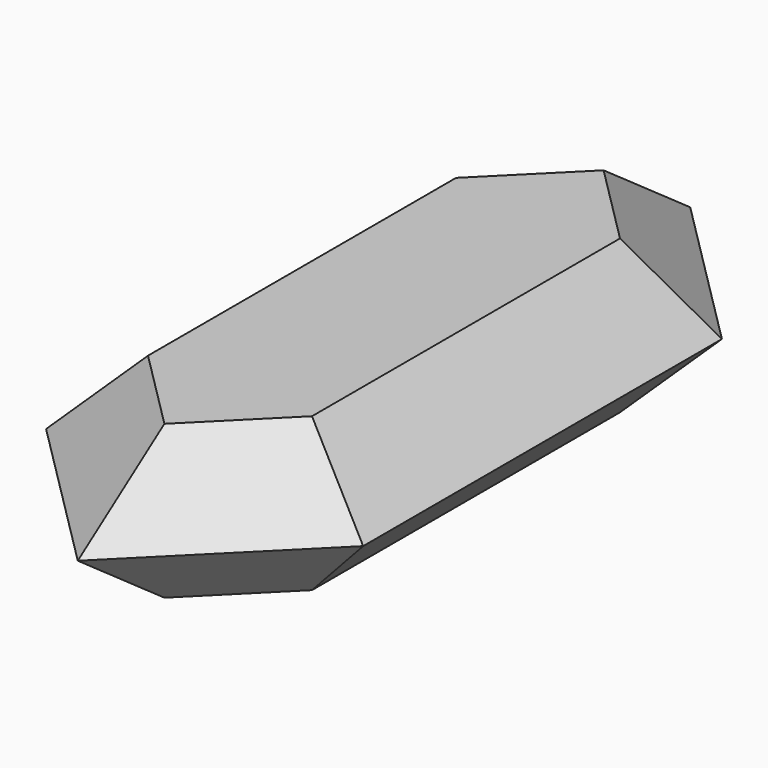
from build123d import *

# Parameters (mm, degrees)
F1_DEPTH = 6
F2_SIZE  = 2.99999


# Not quite as in the source:
# - a fillet or chamfer is up to 0.001 mm smaller than in the source, because OpenCascade refuses the exact size


with BuildPart() as f1:
    # F0 (on Top) → F1 (new body)
    with BuildSketch(Plane.XY):
        Polygon((-6.2132034356, 8.7867965644), (-6.2132034356, 0), (-6.2132034356, -8.7867965644), (0, -15), (6.2132034356, -8.7867965644), (6.2132034356, 0), (6.2132034356, 8.7867965644), (0, 15), align=None)
    extrude(amount=F1_DEPTH)

    # F2 (size 3 in the source; OpenCascade refuses exactly that, so slightly less here)
    f2_edges = [f1.edges().sort_by_distance(p)[0] for p in [
        (-3.106602, 11.893398, 6),
        (3.106602, 11.893398, 6),
        (6.213203, 0, 6),
        (-6.213203, 0, 6),
        (-3.106602, -11.893398, 6),
        (3.106602, -11.893398, 6),
        (-3.106602, 11.893398, 0),
        (-6.213203, 0, 0),
        (-3.106602, -11.893398, 0),
        (3.106602, -11.893398, 0),
        (6.213203, 0, 0),
        (3.106602, 11.893398, 0),
    ]]
    chamfer(f2_edges, length=F2_SIZE)


solid = f1.part
